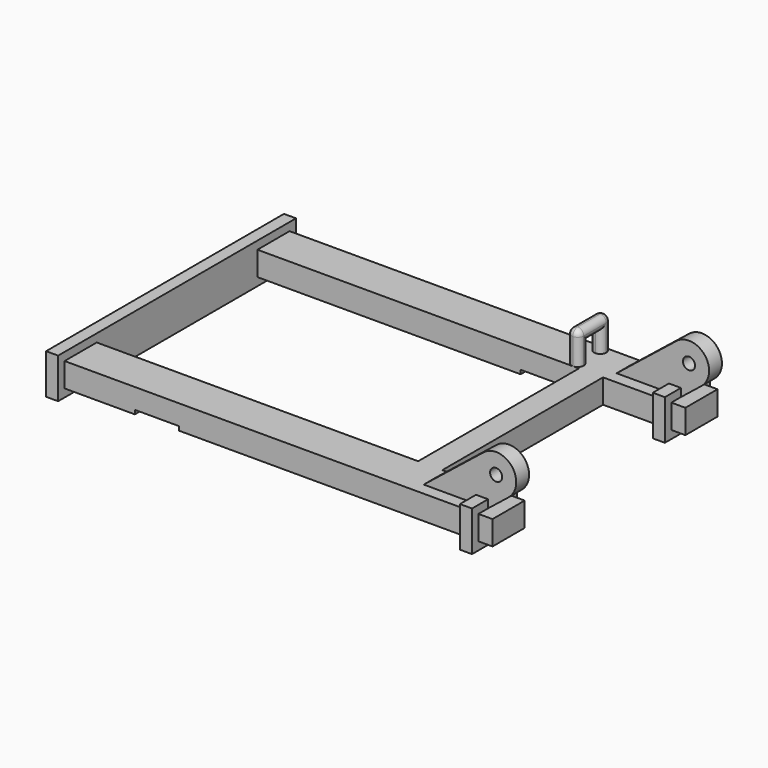
from build123d import *

# Parameters (mm, degrees)
F0_W          = 1.524
F0_H          = 12.7
F1_DEPTH      = 1.524
F2_W          = 0.762
F2_H          = 18.796
F2_H_2        = 3.556
F3_DEPTH      = 0.508
F3_DEPTH_BACK = 2.032
F4_R          = 0.381
F5_DEPTH      = 1.778
F7_DEPTH      = 0.762
F9_W          = 2.794
F9_H          = 2.54
F10_DEPTH     = 0.254
F11_W         = 2.54
F11_H         = 1.524
F12_DEPTH     = 0.889
F13_W         = 2.54
F13_H         = 1.524
F14_DEPTH     = 0.889
F15_W         = 0.762
F15_H         = 0.762
F16_DEPTH     = 2.032
F17_W         = 0.762
F17_H         = 0.762
F18_DEPTH     = 1.016
F19_R         = 0.38099


# Not quite as in the source:
# - a fillet or chamfer is up to 0.001 mm smaller than in the source, because OpenCascade refuses the exact size
# - a pattern or mirror of a feature is missing from the dataset's text; its kind, count and spacing are read off the source's solid


with BuildPart() as f1:
    # F0 (on Top) → F1 (new body)
    with BuildSketch(Plane.XY):
        Polygon((-12.7, 17.78), (-12.7, 15.24), (7.62, 15.24), (9.144, 15.24), (12.7, 15.24), (12.7, 17.78), align=None)
        Polygon((-12.7, 0), (-12.7, 2.54), (-12.7, 15.24), (-12.7, 17.78), (-12.7, 18.288), (-13.462, 18.288), (-13.462, -0.508), (-12.7, -0.508), align=None)
        Polygon((7.62, 2.54), (-12.7, 2.54), (-12.7, 0), (12.7, 0), (12.7, 2.54), (9.144, 2.54), align=None)
        with Locations((8.382, 8.89)):
            Rectangle(F0_W, F0_H)
        Polygon((12.7, 2.54), (12.7, 0), (12.7, -0.508), (13.462, -0.508), (13.462, 3.048), (12.7, 3.048), align=None)
        Polygon((12.7, 18.288), (12.7, 17.78), (12.7, 15.24), (12.7, 14.732), (13.462, 14.732), (13.462, 18.288), align=None)
    extrude(amount=F1_DEPTH)

    # F2 (on face) → F3 (join, two sides)
    with BuildSketch(Plane.XY.offset(1.524)) as f3_sk:
        with Locations((-13.081, 8.89)):
            Rectangle(F2_W, F2_H)
        with Locations((13.081, 16.51)):
            Rectangle(F2_W, F2_H_2)
        with Locations((13.081, 1.27)):
            Rectangle(F2_W, F2_H_2)
    extrude(amount=F3_DEPTH)
    extrude(f3_sk.sketch, amount=-F3_DEPTH_BACK)

    # F4 (on face) → F5 (join)
    with BuildSketch(Plane.XZ):
        with BuildLine():
            Line((13.462, 1.524), (14.762993756, 2.564001561))
            ThreePointArc((14.762993756, 2.564001561), (14.961998439, 4.348993756), (13.177006244, 4.547998439))
            Line((13.177006244, 4.547998439), (9.3941243381, 1.524))
            Line((9.3941243381, 1.524), (13.462, 1.524))
        make_face()
        with Locations((13.97, 3.556)):
            Circle(F4_R, mode=Mode.SUBTRACT)
    f5 = extrude(amount=-F5_DEPTH)

    # F5_copies: F5 across plane
    add(f5.mirror(Plane.ZX.offset(8.89)))

    # F6 (on face) → F7 (cut)
    with BuildSketch(Plane.XZ):
        with BuildLine():
            Line((13.177006244, 4.547998439), (9.3941243381, 1.524))
            Line((9.3941243381, 1.524), (12.7, 1.524))
            Line((12.7, 1.524), (12.7, 2.032))
            Line((12.7, 2.032), (13.462, 2.032))
            Line((13.462, 2.032), (13.462, 1.524))
            Line((13.462, 1.524), (14.762993756, 2.564001561))
            ThreePointArc((14.762993756, 2.564001561), (14.961998439, 4.348993756), (13.177006244, 4.547998439))
        make_face()
    f7 = extrude(amount=-F7_DEPTH, mode=Mode.SUBTRACT)

    # F7_copies: F7 across plane
    add(f7.mirror(Plane.ZX.offset(8.89)), mode=Mode.SUBTRACT)

    # F9 (on face) → F10 (cut)
    with BuildSketch(Plane(origin=(0, 0, 0), x_dir=(1, 0, 0), z_dir=(0, 0, -1))):
        with Locations((5.334, -16.51)):
            Rectangle(F9_W, F9_H)
        with Locations((-6.858, -1.27)):
            Rectangle(F9_W, F9_H)
    extrude(amount=-F10_DEPTH, mode=Mode.SUBTRACT)

    # F11 (on face) → F12 (join)
    with BuildSketch(Plane.YZ.offset(13.462)):
        with Locations((1.27, 0.762)):
            Rectangle(F11_W, F11_H)
    extrude(amount=F12_DEPTH)

    # F13 (on face) → F14 (join)
    with BuildSketch(Plane.YZ.offset(13.462)):
        with Locations((16.51, 0.762)):
            Rectangle(F13_W, F13_H)
    extrude(amount=F14_DEPTH)

    # F15 (on face) → F16 (join)
    with BuildSketch(Plane.XY.offset(1.524)):
        with Locations((7.239, 15.621)):
            Rectangle(F15_W, F15_H)
        with Locations((7.239, 17.399)):
            Rectangle(F15_W, F15_H)
    extrude(amount=F16_DEPTH)

    # F17 (on face) → F18 (join, through all)
    with BuildSketch(Plane.XZ.offset(-17.018)):
        with Locations((7.239, 3.175)):
            Rectangle(F17_W, F17_H)
    extrude(amount=F18_DEPTH)

    # F19 (radius 0.381 in the source; OpenCascade refuses exactly that, so slightly less here)
    f19_edges = [f1.edges().sort_by_distance(p)[0] for p in [
        (6.858, 17.78, 2.54),
        (7.62, 17.78, 2.54),
        (7.239, 17.78, 3.556),
        (6.858, 16.51, 3.556),
        (7.62, 16.51, 3.556),
        (6.858, 17.018, 2.159),
        (6.858, 16.51, 2.794),
        (6.858, 16.002, 2.159),
        (6.858, 15.24, 2.54),
        (7.239, 15.24, 3.556),
        (7.62, 17.018, 2.159),
        (7.62, 16.51, 2.794),
        (7.62, 16.002, 2.159),
        (7.62, 15.24, 2.54),
    ]]
    fillet(f19_edges, radius=F19_R)


solid = f1.part
